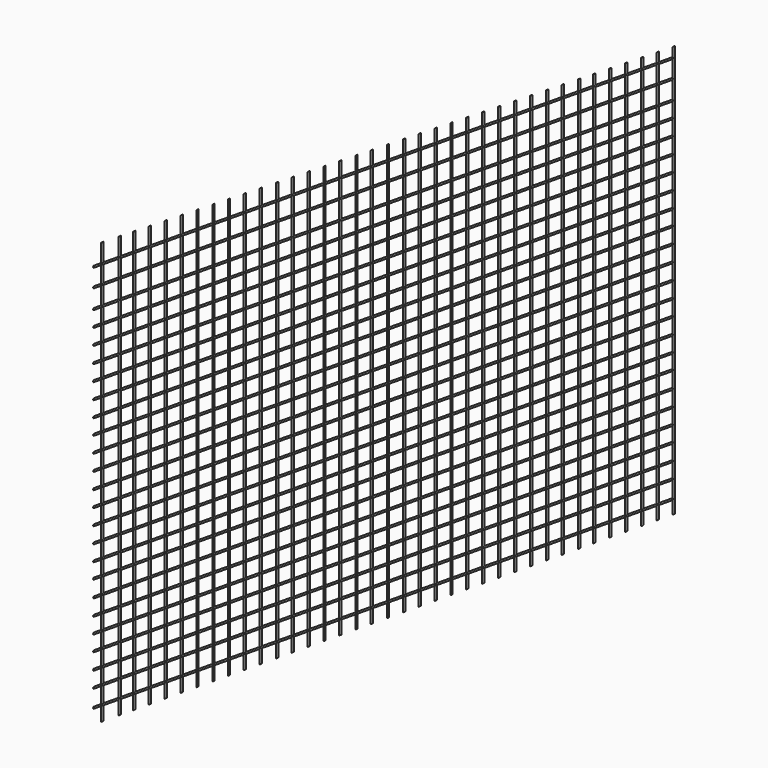
from build123d import *

# Parameters (mm, degrees)
F1_R     = 1.5
F2_DEPTH = 2000
F4_R     = 1.5
F7_DEPTH = 500


with BuildPart() as f2:
    # F1 (on Top) → F2 (new body)
    with BuildSketch(Plane.XY):
        with Locations((34.2302210629, 0)):
            Circle(F1_R)
    extrude(amount=F2_DEPTH)


with BuildPart() as f2b:
    # F1 (on Top) → F2, piece 2 (new body)
    with BuildSketch(Plane.XY):
        with Locations((57.2037696838, 0)):
            Circle(F1_R)
    extrude(amount=F2_DEPTH)


with BuildPart() as f2c:
    # F1 (on Top) → F2, piece 3 (new body)
    with BuildSketch(Plane.XY):
        with Locations((85.0169658661, 0)):
            Circle(F1_R)
    extrude(amount=F2_DEPTH)


with BuildPart() as f2d:
    # F1 (on Top) → F2, piece 4 (new body)
    with BuildSketch(Plane.XY):
        with Locations((107.4634939432, 0)):
            Circle(F1_R)
    extrude(amount=F2_DEPTH)


with BuildPart() as f2e:
    # F1 (on Top) → F2, piece 5 (new body)
    with BuildSketch(Plane.XY):
        with Locations((132.1546733379, 0)):
            Circle(F1_R)
    extrude(amount=F2_DEPTH)


with BuildPart() as f2f:
    # F1 (on Top) → F2, piece 6 (new body)
    with BuildSketch(Plane.XY):
        with Locations((156.8458527327, 0)):
            Circle(F1_R)
    extrude(amount=F2_DEPTH)


with BuildPart() as f2g:
    # F1 (on Top) → F2, piece 7 (new body)
    with BuildSketch(Plane.XY):
        with Locations((182.2104305029, 0)):
            Circle(F1_R)
    extrude(amount=F2_DEPTH)


with BuildPart() as f2h:
    # F1 (on Top) → F2, piece 8 (new body)
    with BuildSketch(Plane.XY):
        with Locations((207.1260809898, 0)):
            Circle(F1_R)
    extrude(amount=F2_DEPTH)


with BuildPart() as f2i:
    # F1 (on Top) → F2, piece 9 (new body)
    with BuildSketch(Plane.XY):
        with Locations((232.2661876678, 0)):
            Circle(F1_R)
    extrude(amount=F2_DEPTH)


with BuildPart() as f2j:
    # F1 (on Top) → F2, piece 10 (new body)
    with BuildSketch(Plane.XY):
        with Locations((256.7329108715, 0)):
            Circle(F1_R)
    extrude(amount=F2_DEPTH)


with BuildPart() as f2k:
    # F1 (on Top) → F2, piece 11 (new body)
    with BuildSketch(Plane.XY):
        with Locations((281.6485464573, 0)):
            Circle(F1_R)
    extrude(amount=F2_DEPTH)


with BuildPart() as f2l:
    # F1 (on Top) → F2, piece 12 (new body)
    with BuildSketch(Plane.XY):
        with Locations((307.0131242275, 0)):
            Circle(F1_R)
    extrude(amount=F2_DEPTH)


with BuildPart() as f2m:
    # F1 (on Top) → F2, piece 13 (new body)
    with BuildSketch(Plane.XY):
        with Locations((332.3777318001, 0)):
            Circle(F1_R)
    extrude(amount=F2_DEPTH)


with BuildPart() as f2n:
    # F1 (on Top) → F2, piece 14 (new body)
    with BuildSketch(Plane.XY):
        with Locations((357.2933673859, 0)):
            Circle(F1_R)
    extrude(amount=F2_DEPTH)


with BuildPart() as f2o:
    # F1 (on Top) → F2, piece 15 (new body)
    with BuildSketch(Plane.XY):
        with Locations((381.9845318794, 0)):
            Circle(F1_R)
    extrude(amount=F2_DEPTH)


with BuildPart() as f2p:
    # F1 (on Top) → F2, piece 16 (new body)
    with BuildSketch(Plane.XY):
        with Locations((407.0443809032, 0)):
            Circle(F1_R)
    extrude(amount=F2_DEPTH)


with BuildPart() as f2q:
    # F1 (on Top) → F2, piece 17 (new body)
    with BuildSketch(Plane.XY):
        with Locations((432.1222901344, 0)):
            Circle(F1_R)
    extrude(amount=F2_DEPTH)


with BuildPart() as f2r:
    # F1 (on Top) → F2, piece 18 (new body)
    with BuildSketch(Plane.XY):
        with Locations((457.5176239014, 0)):
            Circle(F1_R)
    extrude(amount=F2_DEPTH)


with BuildPart() as f2s:
    # F1 (on Top) → F2, piece 19 (new body)
    with BuildSketch(Plane.XY):
        with Locations((481.643229723, 0)):
            Circle(F1_R)
    extrude(amount=F2_DEPTH)


with BuildPart() as f2t:
    # F1 (on Top) → F2, piece 20 (new body)
    with BuildSketch(Plane.XY):
        with Locations((507.0385932922, 0)):
            Circle(F1_R)
    extrude(amount=F2_DEPTH)


with BuildPart() as f2u:
    # F1 (on Top) → F2, piece 21 (new body)
    with BuildSketch(Plane.XY):
        with Locations((532.4339270592, 0)):
            Circle(F1_R)
    extrude(amount=F2_DEPTH)


with BuildPart() as f2v:
    # F1 (on Top) → F2, piece 22 (new body)
    with BuildSketch(Plane.XY):
        with Locations((557.1944117546, 0)):
            Circle(F1_R)
    extrude(amount=F2_DEPTH)


with BuildPart() as f2w:
    # F1 (on Top) → F2, piece 23 (new body)
    with BuildSketch(Plane.XY):
        with Locations((581.9548368454, 0)):
            Circle(F1_R)
    extrude(amount=F2_DEPTH)


with BuildPart() as f2x:
    # F1 (on Top) → F2, piece 24 (new body)
    with BuildSketch(Plane.XY):
        with Locations((607.0327758789, 0)):
            Circle(F1_R)
    extrude(amount=F2_DEPTH)


with BuildPart() as f2y:
    # F1 (on Top) → F2, piece 25 (new body)
    with BuildSketch(Plane.XY):
        with Locations((632.1106553078, 0)):
            Circle(F1_R)
    extrude(amount=F2_DEPTH)


with BuildPart() as f2z:
    # F1 (on Top) → F2, piece 26 (new body)
    with BuildSketch(Plane.XY):
        with Locations((657.1885347366, 0)):
            Circle(F1_R)
    extrude(amount=F2_DEPTH)


with BuildPart() as f2ba:
    # F1 (on Top) → F2, piece 27 (new body)
    with BuildSketch(Plane.XY):
        with Locations((682.2664737701, 0)):
            Circle(F1_R)
    extrude(amount=F2_DEPTH)


with BuildPart() as f2bb:
    # F1 (on Top) → F2, piece 28 (new body)
    with BuildSketch(Plane.XY):
        with Locations((707.6618075371, 0)):
            Circle(F1_R)
    extrude(amount=F2_DEPTH)


with BuildPart() as f2bc:
    # F1 (on Top) → F2, piece 29 (new body)
    with BuildSketch(Plane.XY):
        with Locations((732.7397465706, 0)):
            Circle(F1_R)
    extrude(amount=F2_DEPTH)


with BuildPart() as f2bd:
    # F1 (on Top) → F2, piece 30 (new body)
    with BuildSketch(Plane.XY):
        with Locations((757.5001716614, 0)):
            Circle(F1_R)
    extrude(amount=F2_DEPTH)


with BuildPart() as f2be:
    # F1 (on Top) → F2, piece 31 (new body)
    with BuildSketch(Plane.XY):
        with Locations((782.2606563568, 0)):
            Circle(F1_R)
    extrude(amount=F2_DEPTH)


with BuildPart() as f2bf:
    # F1 (on Top) → F2, piece 32 (new body)
    with BuildSketch(Plane.XY):
        with Locations((807.9734444618, 0)):
            Circle(F1_R)
    extrude(amount=F2_DEPTH)


with BuildPart() as f2bg:
    # F1 (on Top) → F2, piece 33 (new body)
    with BuildSketch(Plane.XY):
        with Locations((832.147538662, 0)):
            Circle(F1_R)
    extrude(amount=F2_DEPTH)


with BuildPart() as f2bh:
    # F1 (on Top) → F2, piece 34 (new body)
    with BuildSketch(Plane.XY):
        with Locations((857.1060299873, 0)):
            Circle(F1_R)
    extrude(amount=F2_DEPTH)


with BuildPart() as f2bi:
    # F1 (on Top) → F2, piece 35 (new body)
    with BuildSketch(Plane.XY):
        with Locations((882.4648857117, 0)):
            Circle(F1_R)
    extrude(amount=F2_DEPTH)


with BuildPart() as f2bj:
    # F1 (on Top) → F2, piece 36 (new body)
    with BuildSketch(Plane.XY):
        with Locations((907.2899222374, 0)):
            Circle(F1_R)
    extrude(amount=F2_DEPTH)


with BuildPart() as f2bk:
    # F1 (on Top) → F2, piece 37 (new body)
    with BuildSketch(Plane.XY):
        with Locations((931.9815039635, 0)):
            Circle(F1_R)
    extrude(amount=F2_DEPTH)


with BuildPart() as f2bl:
    # F1 (on Top) → F2, piece 38 (new body)
    with BuildSketch(Plane.XY):
        with Locations((956.8064808846, 0)):
            Circle(F1_R)
    extrude(amount=F2_DEPTH)


with BuildPart() as f5:
    # F5: sweep along a path in F3
    with BuildLine(Plane.XZ) as f5_path:
        Line((0, 145.7352638245), (957.4801921844, 760.9102725983))
    # F4 (on Right) → F5 (sweep)
    with BuildSketch(Plane.YZ):
        with Locations((0, 145.5413401127)):
            Circle(F4_R)
        with Locations((0, 173.2242256403)):
            Circle(F4_R)
        with Locations((0, 198.2319205999)):
            Circle(F4_R)
        with Locations((0, 223.7721383572)):
            Circle(F4_R)
        with Locations((0, 248.3791410923)):
            Circle(F4_R)
        with Locations((0, 272.9861438274)):
            Circle(F4_R)
        with Locations((0, 298.4320223331)):
            Circle(F4_R)
        with Locations((0, 324.4371414185)):
            Circle(F4_R)
        with Locations((0, 348.484903574)):
            Circle(F4_R)
        with Locations((0, 373.3715116978)):
            Circle(F4_R)
        with Locations((0, 398.4470963478)):
            Circle(F4_R)
        with Locations((0, 423.6133396626)):
            Circle(F4_R)
        with Locations((0, 448.4261572361)):
            Circle(F4_R)
        with Locations((0, 473.8208055496)):
            Circle(F4_R)
        with Locations((0, 498.9803433418)):
            Circle(F4_R)
        with Locations((0, 523.9047408104)):
            Circle(F4_R)
        with Locations((0, 548.123717308)):
            Circle(F4_R)
        with Locations((0, 573.048055172)):
            Circle(F4_R)
        with Locations((0, 598.2075929642)):
            Circle(F4_R)
        with Locations((0, 623.2078671455)):
            Circle(F4_R)
        with Locations((0, 648.5166549683)):
            Circle(F4_R)
        with Locations((0, 673.4299659729)):
            Circle(F4_R)
        with Locations((0, 698.1455683708)):
            Circle(F4_R)
        with Locations((0, 728.243470192)):
            Circle(F4_R)
        with Locations((0, 756.8411827087)):
            Circle(F4_R)
    sweep(path=f5_path.line)


with BuildPart() as f7_tool:
    # F6 (on Front) → F7 (new body, symmetric)
    with BuildSketch(Plane.XZ):
        Polygon((-23.6240005611, 816.5537986777), (-13.3388005197, 779.176235199), (44.032342732, 815.1211429726), (44.032342732, 870.409488678), align=None)
        Polygon((44.032342732, 815.1211429726), (-13.3388005197, 779.176235199), (-23.6240005611, 816.5537986777), (-128.896817565, 68.474188447), (-30.5964027953, 68.474188447), (0, 122.276738286), (44.032342732, 150.6478036303), align=None)
        Polygon((44.032342732, 870.409488678), (44.032342732, 815.1211429726), (1253.7178993225, 1573.028922081), (1173.9851236343, 2220.8743095398), (-382.9669952393, 2122.4462985992), (-23.6240005611, 816.5537986777), align=None)
        Polygon((44.032342732, 68.474188447), (44.032342732, 150.6478036303), (0, 122.276738286), (-30.5964027953, 68.474188447), align=None)
        Polygon((1642.1811580658, 1180.3723573685), (44.032342732, 150.6478036303), (44.032342732, 68.474188447), (-30.5964027953, 68.474188447), (-129.7628283501, -105.9060022235), (1406.7068099976, -73.5282897949), align=None)
    extrude(amount=F7_DEPTH, both=True)


with BuildPart() as f2_1:
    add(f2.part)

    # F7: cut by f7_tool
    add(f7_tool.part, mode=Mode.SUBTRACT)


with BuildPart() as f2b_1:
    add(f2b.part)

    # F7: cut by f7_tool
    add(f7_tool.part, mode=Mode.SUBTRACT)


with BuildPart() as f2c_1:
    add(f2c.part)

    # F7: cut by f7_tool
    add(f7_tool.part, mode=Mode.SUBTRACT)


with BuildPart() as f2d_1:
    add(f2d.part)

    # F7: cut by f7_tool
    add(f7_tool.part, mode=Mode.SUBTRACT)


with BuildPart() as f2e_1:
    add(f2e.part)

    # F7: cut by f7_tool
    add(f7_tool.part, mode=Mode.SUBTRACT)


with BuildPart() as f2f_1:
    add(f2f.part)

    # F7: cut by f7_tool
    add(f7_tool.part, mode=Mode.SUBTRACT)


with BuildPart() as f2g_1:
    add(f2g.part)

    # F7: cut by f7_tool
    add(f7_tool.part, mode=Mode.SUBTRACT)


with BuildPart() as f2h_1:
    add(f2h.part)

    # F7: cut by f7_tool
    add(f7_tool.part, mode=Mode.SUBTRACT)


with BuildPart() as f2i_1:
    add(f2i.part)

    # F7: cut by f7_tool
    add(f7_tool.part, mode=Mode.SUBTRACT)


with BuildPart() as f2j_1:
    add(f2j.part)

    # F7: cut by f7_tool
    add(f7_tool.part, mode=Mode.SUBTRACT)


with BuildPart() as f2k_1:
    add(f2k.part)

    # F7: cut by f7_tool
    add(f7_tool.part, mode=Mode.SUBTRACT)


with BuildPart() as f2l_1:
    add(f2l.part)

    # F7: cut by f7_tool
    add(f7_tool.part, mode=Mode.SUBTRACT)


with BuildPart() as f2m_1:
    add(f2m.part)

    # F7: cut by f7_tool
    add(f7_tool.part, mode=Mode.SUBTRACT)


with BuildPart() as f2n_1:
    add(f2n.part)

    # F7: cut by f7_tool
    add(f7_tool.part, mode=Mode.SUBTRACT)


with BuildPart() as f2o_1:
    add(f2o.part)

    # F7: cut by f7_tool
    add(f7_tool.part, mode=Mode.SUBTRACT)


with BuildPart() as f2p_1:
    add(f2p.part)

    # F7: cut by f7_tool
    add(f7_tool.part, mode=Mode.SUBTRACT)


with BuildPart() as f2q_1:
    add(f2q.part)

    # F7: cut by f7_tool
    add(f7_tool.part, mode=Mode.SUBTRACT)


with BuildPart() as f2r_1:
    add(f2r.part)

    # F7: cut by f7_tool
    add(f7_tool.part, mode=Mode.SUBTRACT)


with BuildPart() as f2s_1:
    add(f2s.part)

    # F7: cut by f7_tool
    add(f7_tool.part, mode=Mode.SUBTRACT)


with BuildPart() as f2t_1:
    add(f2t.part)

    # F7: cut by f7_tool
    add(f7_tool.part, mode=Mode.SUBTRACT)


with BuildPart() as f2u_1:
    add(f2u.part)

    # F7: cut by f7_tool
    add(f7_tool.part, mode=Mode.SUBTRACT)


with BuildPart() as f2v_1:
    add(f2v.part)

    # F7: cut by f7_tool
    add(f7_tool.part, mode=Mode.SUBTRACT)


with BuildPart() as f2w_1:
    add(f2w.part)

    # F7: cut by f7_tool
    add(f7_tool.part, mode=Mode.SUBTRACT)


with BuildPart() as f2x_1:
    add(f2x.part)

    # F7: cut by f7_tool
    add(f7_tool.part, mode=Mode.SUBTRACT)


with BuildPart() as f2y_1:
    add(f2y.part)

    # F7: cut by f7_tool
    add(f7_tool.part, mode=Mode.SUBTRACT)


with BuildPart() as f2z_1:
    add(f2z.part)

    # F7: cut by f7_tool
    add(f7_tool.part, mode=Mode.SUBTRACT)


with BuildPart() as f2ba_1:
    add(f2ba.part)

    # F7: cut by f7_tool
    add(f7_tool.part, mode=Mode.SUBTRACT)


with BuildPart() as f2bb_1:
    add(f2bb.part)

    # F7: cut by f7_tool
    add(f7_tool.part, mode=Mode.SUBTRACT)


with BuildPart() as f2bc_1:
    add(f2bc.part)

    # F7: cut by f7_tool
    add(f7_tool.part, mode=Mode.SUBTRACT)


with BuildPart() as f2bd_1:
    add(f2bd.part)

    # F7: cut by f7_tool
    add(f7_tool.part, mode=Mode.SUBTRACT)


with BuildPart() as f2be_1:
    add(f2be.part)

    # F7: cut by f7_tool
    add(f7_tool.part, mode=Mode.SUBTRACT)


with BuildPart() as f2bf_1:
    add(f2bf.part)

    # F7: cut by f7_tool
    add(f7_tool.part, mode=Mode.SUBTRACT)


with BuildPart() as f2bg_1:
    add(f2bg.part)

    # F7: cut by f7_tool
    add(f7_tool.part, mode=Mode.SUBTRACT)


with BuildPart() as f2bh_1:
    add(f2bh.part)

    # F7: cut by f7_tool
    add(f7_tool.part, mode=Mode.SUBTRACT)


with BuildPart() as f2bi_1:
    add(f2bi.part)

    # F7: cut by f7_tool
    add(f7_tool.part, mode=Mode.SUBTRACT)


with BuildPart() as f2bj_1:
    add(f2bj.part)

    # F7: cut by f7_tool
    add(f7_tool.part, mode=Mode.SUBTRACT)


with BuildPart() as f2bk_1:
    add(f2bk.part)

    # F7: cut by f7_tool
    add(f7_tool.part, mode=Mode.SUBTRACT)


with BuildPart() as f2bl_1:
    add(f2bl.part)

    # F7: cut by f7_tool
    add(f7_tool.part, mode=Mode.SUBTRACT)


with BuildPart() as f5_1:
    add(f5.part)

    # F7: cut by f7_tool
    add(f7_tool.part, mode=Mode.SUBTRACT)


solid = Compound([f2b_1.part, f2c_1.part, f2d_1.part, f2e_1.part, f2f_1.part, f2g_1.part, f2h_1.part, f2i_1.part, f2j_1.part, f2k_1.part, f2l_1.part, f2m_1.part, f2n_1.part, f2o_1.part, f2p_1.part, f2q_1.part, f2r_1.part, f2s_1.part, f2t_1.part, f2u_1.part, f2v_1.part, f2w_1.part, f2x_1.part, f2y_1.part, f2z_1.part, f2ba_1.part, f2bb_1.part, f2bc_1.part, f2bd_1.part, f2be_1.part, f2bf_1.part, f2bg_1.part, f2bh_1.part, f2bi_1.part, f2bj_1.part, f2bk_1.part, f2bl_1.part, f5_1.part])
